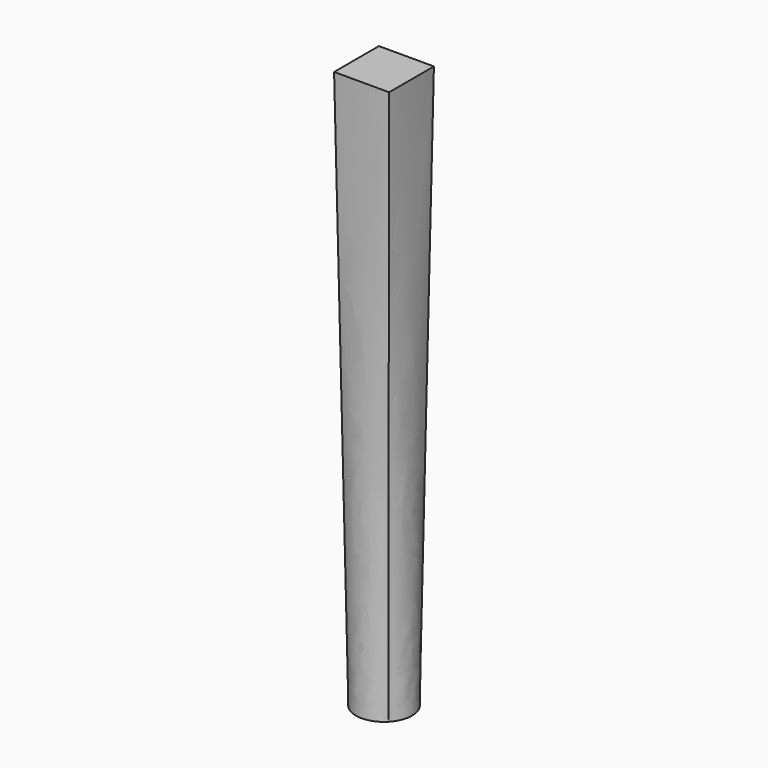
from build123d import *

# Parameters (mm, degrees)
F0_W     = 50
F0_H     = 50
F1_DEPTH = 500
F5_W     = 49.1124280814
F5_H     = 50


# Not quite as in the source:
# - the arcs of a loft's sections are written as splines that run evenly, so that the points pair up as in the source's solid


with BuildPart() as f1:
    # F0 (on Top) → F1 (new body)
    with BuildSketch(Plane.XY):
        with Locations((-40.0555571541, -0.6388908335)):
            Rectangle(F0_W, F0_H)
    extrude(amount=F1_DEPTH)


with BuildPart() as f6:
    # F3 (on Top) → F6 section 0
    with BuildSketch(Plane.XY):
        with BuildLine():
            add(Edge.make_bspline(
                [(17.5186599633, 17.8352615088), (16.3513448273, 18.9818551222), (15.0711317337, 20.0134527208), (12.3339820931, 21.8071132264), (10.8771132275, 22.5691317816), (7.8426313441, 23.7943361988), (6.2650933599, 24.2574917651), (3.0498926708, 24.8671561751), (1.412309468, 25.0136499437), (-1.8600516675, 24.9843452853), (-3.4947486847, 24.8085475829), (-6.6985152634, 24.1414000176), (-8.2675056054, 23.6500666512), (-11.2795586742, 22.3707142858), (-12.7225469221, 21.5827269212), (-15.4271349709, 19.7403345496), (-16.6886678955, 18.6859750994), (-17.8352615088, 17.5186599633)],
                knots=[0, 0, 0, 0, 0.125, 0.125, 0.25, 0.25, 0.375, 0.375, 0.5, 0.5, 0.625, 0.625, 0.75, 0.75, 0.875, 0.875, 1, 1, 1, 1], degree=3))
            add(Edge.make_bspline(
                [(-17.8352615088, 17.5186599633), (-18.9818551222, 16.3513448273), (-20.0134527208, 15.0711317337), (-21.8071132264, 12.3339820931), (-22.5691317816, 10.8771132275), (-23.7943361988, 7.8426313441), (-24.2574917651, 6.2650933599), (-24.8671561751, 3.0498926708), (-25.0136499437, 1.412309468), (-24.9843452853, -1.8600516675), (-24.8085475829, -3.4947486847), (-24.1414000176, -6.6985152634), (-23.6500666512, -8.2675056054), (-22.3707142858, -11.2795586742), (-21.5827269212, -12.7225469221), (-19.7403345496, -15.4271349709), (-18.6859750994, -16.6886678955), (-17.5186599633, -17.8352615088)],
                knots=[0, 0, 0, 0, 0.125, 0.125, 0.25, 0.25, 0.375, 0.375, 0.5, 0.5, 0.625, 0.625, 0.75, 0.75, 0.875, 0.875, 1, 1, 1, 1], degree=3))
            add(Edge.make_bspline(
                [(-17.5186599633, -17.8352615088), (-16.3513448273, -18.9818551222), (-15.0711317337, -20.0134527208), (-12.3339820931, -21.8071132264), (-10.8771132275, -22.5691317816), (-7.8426313441, -23.7943361988), (-6.2650933599, -24.2574917651), (-3.0498926708, -24.8671561751), (-1.412309468, -25.0136499437), (1.8600516675, -24.9843452853), (3.4947486847, -24.8085475829), (6.6985152634, -24.1414000176), (8.2675056054, -23.6500666512), (11.2795586742, -22.3707142858), (12.7225469221, -21.5827269212), (15.4271349709, -19.7403345496), (16.6886678955, -18.6859750994), (17.8352615088, -17.5186599633)],
                knots=[0, 0, 0, 0, 0.125, 0.125, 0.25, 0.25, 0.375, 0.375, 0.5, 0.5, 0.625, 0.625, 0.75, 0.75, 0.875, 0.875, 1, 1, 1, 1], degree=3))
            add(Edge.make_bspline(
                [(17.8352615088, -17.5186599633), (18.9818551222, -16.3513448273), (20.0134527208, -15.0711317337), (21.8071132264, -12.3339820931), (22.5691317816, -10.8771132275), (23.7943361988, -7.8426313441), (24.2574917651, -6.2650933599), (24.8671561751, -3.0498926708), (25.0136499437, -1.412309468), (24.9843452853, 1.8600516675), (24.8085475829, 3.4947486847), (24.1414000176, 6.6985152634), (23.6500666512, 8.2675056054), (22.3707142858, 11.2795586742), (21.5827269212, 12.7225469221), (19.7403345496, 15.4271349709), (18.6859750994, 16.6886678955), (17.5186599633, 17.8352615088)],
                knots=[0, 0, 0, 0, 0.125, 0.125, 0.25, 0.25, 0.375, 0.375, 0.5, 0.5, 0.625, 0.625, 0.75, 0.75, 0.875, 0.875, 1, 1, 1, 1], degree=3))
        make_face()
    # F5 (on offset) → F6 section 1
    with BuildSketch(Plane.XY.offset(500)):
        Rectangle(F5_W, F5_H)
    loft(ruled=True)


solid = f6.part
